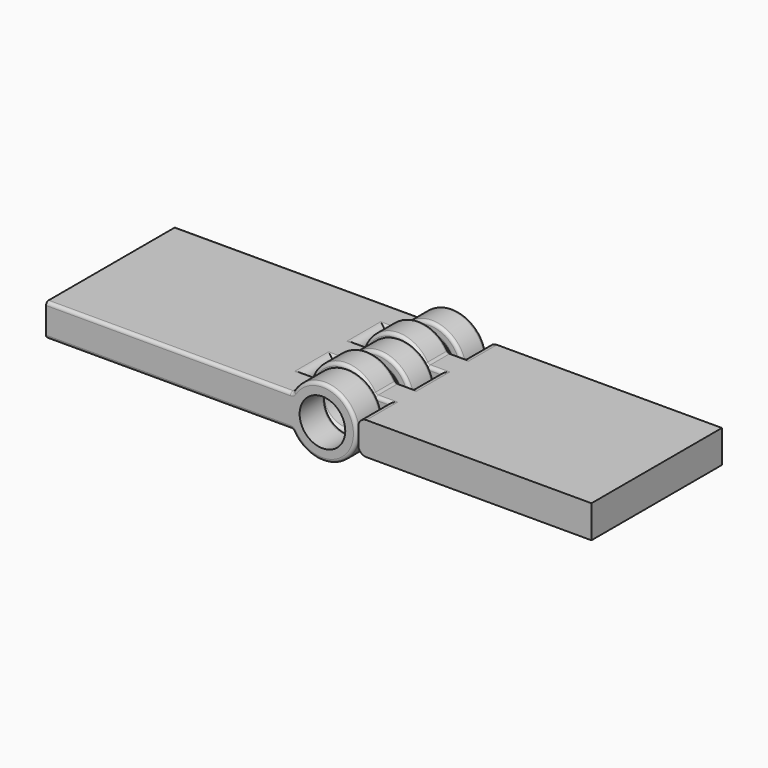
from build123d import *

# Parameters (mm, degrees)
F1_DEPTH      = 50
F1_DEPTH_BACK = 50
F2_R          = 14
F2_R_2        = 10
F3_DEPTH      = 25
F3_DEPTH_BACK = 160.8
F6_W          = 41.9630929828
F6_H          = 20
F7_DEPTH      = 25
F7_DEPTH_BACK = 25
F6_W_2        = 41.4589837193
F8_DEPTH      = 32
F8_DEPTH_BACK = 48
F10_DEPTH     = 8
F11_DEPTH     = 8
F12_DEPTH     = 2
F13_DEPTH     = 2
F14_R         = 5
F14_2_R       = 5
F15_R         = 2
F15_2_R       = 2


# Not quite as in the source:
# - two fillets or chamfers of one size are made in one step
# - a feature of the source that left no trace in its solid (it failed there, or was rolled back) is left out
# - a feature names something its author has since deleted; it is built from what else it names


with BuildPart() as f1:
    # F0 (on Front) → F1 (new body, two sides)
    with BuildSketch(Plane.XZ) as f1_sk:
        with BuildLine():
            Line((76.7551469592, -10), (58.2889616489, -10))
            ThreePointArc((58.2889616489, -10), (76.7551469616, -21), (95.2213322742, -10))
            Line((95.2213322742, -10), (76.7551469592, -10))
        make_face()
        with BuildLine():
            Line((-92.7030667663, -10), (58.2889616489, -10))
            Line((58.2889616489, -10), (76.7551469592, -10))
            ThreePointArc((76.7551469592, -10), (66.7551469616, 2.4e-09), (76.755146964, 10))
            Line((76.755146964, 10), (58.2889616489, 10))
            Line((58.2889616489, 10), (-92.7030667663, 10))
            Line((-92.7030667663, 10), (-92.7030667663, -10))
        make_face()
        with BuildLine():
            Line((76.7551469592, -10), (95.2213322742, -10))
            ThreePointArc((95.2213322742, -10), (86.7551469616, 18.4661853126), (58.2889616489, 10))
            Line((58.2889616489, 10), (76.755146964, 10))
            ThreePointArc((76.755146964, 10), (83.8262147743, 7.071067811), (86.7551469616, 0))
            ThreePointArc((86.7551469616, 0), (83.8262147726, -7.0710678127), (76.7551469592, -10))
        make_face()
    extrude(amount=-F1_DEPTH)
    extrude(f1_sk.sketch, amount=F1_DEPTH_BACK)

    # F2 (on face) → F3 (cut, two sides)
    with BuildSketch(Plane.XZ.offset(50)) as f3_sk:
        with Locations((76.7551469616, 0)):
            Circle(F2_R)
        with Locations((76.7551469616, 0)):
            Circle(F2_R_2, mode=Mode.SUBTRACT)
    extrude(amount=F3_DEPTH, mode=Mode.SUBTRACT)
    extrude(f3_sk.sketch, amount=-F3_DEPTH_BACK, mode=Mode.SUBTRACT)


with BuildPart() as f5_1:
    # F5: instance of F1
    add(f1.part.mirror(Plane.YZ.offset(100)))

    # F6 (on Top) → F8 (cut, two sides)
    with BuildSketch(Plane.XY) as f8_sk:
        with Locations((120.9815464914, 40)):
            Rectangle(F6_W_2, F6_H)
        with Locations((120.9815464914, -40)):
            Rectangle(F6_W_2, F6_H)
        with Locations((120.9815464914, 0)):
            Rectangle(F6_W_2, F6_H)
    extrude(amount=F8_DEPTH, mode=Mode.SUBTRACT)
    extrude(f8_sk.sketch, amount=-F8_DEPTH_BACK, mode=Mode.SUBTRACT)


with BuildPart() as f1_1:
    add(f1.part)

    # F6 (on Top) → F7 (cut, two sides)
    with BuildSketch(Plane.XY) as f7_sk:
        with Locations((79.2705081403, 20)):
            Rectangle(F6_W, F6_H)
        with Locations((79.2705081403, -20)):
            Rectangle(F6_W, F6_H)
    extrude(amount=F7_DEPTH, mode=Mode.SUBTRACT)
    extrude(f7_sk.sketch, amount=-F7_DEPTH_BACK, mode=Mode.SUBTRACT)

    # F10 (cut): faces of the model
    f10_faces = [f1_1.faces().sort_by_distance(p)[0] for p in [
        (58.2889616489, -20, 0),
        (58.2889616489, 20, 0),
    ]]
    extrude(f10_faces, amount=-F10_DEPTH, mode=Mode.SUBTRACT)


with BuildPart() as f5_1_1:
    # F9: moved
    add(f5_1.part.moved(Location((-51, 0, 0))))

    # F11 (cut): faces of the model
    f11_faces = [f5_1_1.faces().sort_by_distance(p)[0] for p in [
        (90.7110383511, 40, 0),
        (90.7110383511, 0, 0),
        (90.7110383511, -40, 0),
    ]]
    extrude(f11_faces, amount=-F11_DEPTH, mode=Mode.SUBTRACT)


with BuildPart() as f12_tool:
    # F12 (cut): faces of the model
    f12_faces = [f1_1.part.faces().sort_by_distance(p)[0] for p in [
        (54.2889616489, 30, 9.3661988681),
        (54.2889616489, -10, 9.3661988681),
        (54.2889616489, -30, 9.3661988681),
        (54.2889616489, 10, 9.3661988681),
    ]]
    extrude(f12_faces, amount=-F12_DEPTH, dir=(0, -1, 0))


with BuildPart() as f1_2:
    add(f1_1.part)

    # F12: cut by f12_tool
    add(f12_tool.part, mode=Mode.SUBTRACT)

    # F14
    f14_edges = [f1_2.edges().sort_by_distance(p)[0] for p in [
        (50.288962, -19, -10),
        (50.288962, -19, 10),
        (50.288962, 21, -10),
        (50.288962, 21, 10),
        (58.288962, 41, -10),
        (58.288962, 41, 10),
    ]]
    fillet(f14_edges, radius=F14_R)

    # F15
    f15_edges = [f1_2.edges().sort_by_distance(p)[0] for p in [
        (47.788962, -30, 10),
        (47.788962, -30, -10),
        (54.288962, -30, 10),
        (54.288962, -30, -10),
        (97.755147, -30, 0),
        (62.755147, -30, 0),
        (52.903674, 32, 10),
        (47.788962, 32, 10),
        (-18.59234, 50, 10),
        (47.788962, 10, 10),
        (-17.207053, -50, 10),
        (54.288962, 10, 10),
        (58.288962, -40, 10),
        (58.288962, 1, 10),
        (54.288962, -8, 10),
        (47.788962, -8, 10),
        (-18.59234, 50, -10),
        (52.903674, 32, -10),
        (-17.207053, -50, -10),
        (47.788962, 32, -10),
        (58.288962, -40, -10),
        (47.788962, 10, -10),
        (54.288962, 10, -10),
        (58.288962, 1, -10),
        (47.788962, -8, -10),
        (54.288962, -8, -10),
        (97.755147, -50, 0),
        (97.755147, -8, 0),
        (62.755147, -8, 0),
        (57.818052, 32, 10.560232),
        (97.755147, 32, 0),
        (57.818052, 32, -10.560232),
        (62.755147, 32, 0),
        (57.818052, 50, 10.560232),
        (97.755147, 50, 0),
        (57.818052, 50, -10.560232),
        (62.755147, 50, 0),
        (97.755147, 10, 0),
        (62.755147, 10, 0),
    ]]
    fillet(f15_edges, radius=F15_R)


with BuildPart() as f5_1_2:
    add(f5_1_1.part)

    # F12: cut by f12_tool
    add(f12_tool.part, mode=Mode.SUBTRACT)

    # F13 (cut): faces of the model
    f13_faces = [f5_1_2.faces().sort_by_distance(p)[0] for p in [
        (97.9581686472, -30, 0),
        (86.5686168108, -30, 0),
        (61.3068071178, -30, -15.4798434001),
        (61.3068071178, -30, 15.4798434001),
        (97.9581686472, 10, 0),
        (86.5686168108, 10, 0),
        (61.3068071178, 10, -15.4798434001),
        (61.3068071178, 10, 15.4798434001),
        (94.7110383511, -10, -9.3661988681),
        (94.7110383511, 30, -9.3661988681),
    ]]
    extrude(f13_faces, amount=-F13_DEPTH, dir=(0, -1, 0), mode=Mode.SUBTRACT)

    # F14#2
    f14_2_edges = [f5_1_2.edges().sort_by_distance(p)[0] for p in [
        (98.711038, -39, 10),
        (98.711038, -39, -10),
        (98.711038, 1, -10),
        (98.711038, 1, 10),
        (98.711038, 40, -10),
        (98.711038, 40, 10),
    ]]
    fillet(f14_2_edges, radius=F14_2_R)

    # F15#2
    f15_2_edges = [f5_1_2.edges().sort_by_distance(p)[0] for p in [
        (101.211038, 30, -10),
        (94.711038, 30, -10),
        (90.711038, 21, -10),
        (101.211038, -28, -10),
        (94.711038, 12, -10),
        (94.711038, -28, -10),
        (101.211038, 12, -10),
        (90.711038, -19, -10),
        (94.711038, -10, -10),
        (101.211038, -10, -10),
        (101.211038, 30, 10),
        (94.711038, 30, 10),
        (90.711038, 21, 10),
        (101.211038, -28, 10),
        (94.711038, 12, 10),
        (94.711038, -28, 10),
        (101.211038, 12, 10),
        (90.711038, -19, 10),
        (94.711038, -10, 10),
        (101.211038, -10, 10),
        (51.244853, 30, 0),
        (86.244853, 30, 0),
        (51.244853, 12, 0),
        (51.244853, -28, 0),
        (86.244853, -28, 0),
        (86.244853, 12, 0),
        (51.244853, -10, 0),
        (86.244853, -10, 0),
    ]]
    fillet(f15_2_edges, radius=F15_2_R)


solid = Compound([f1_2.part, f5_1_2.part])
